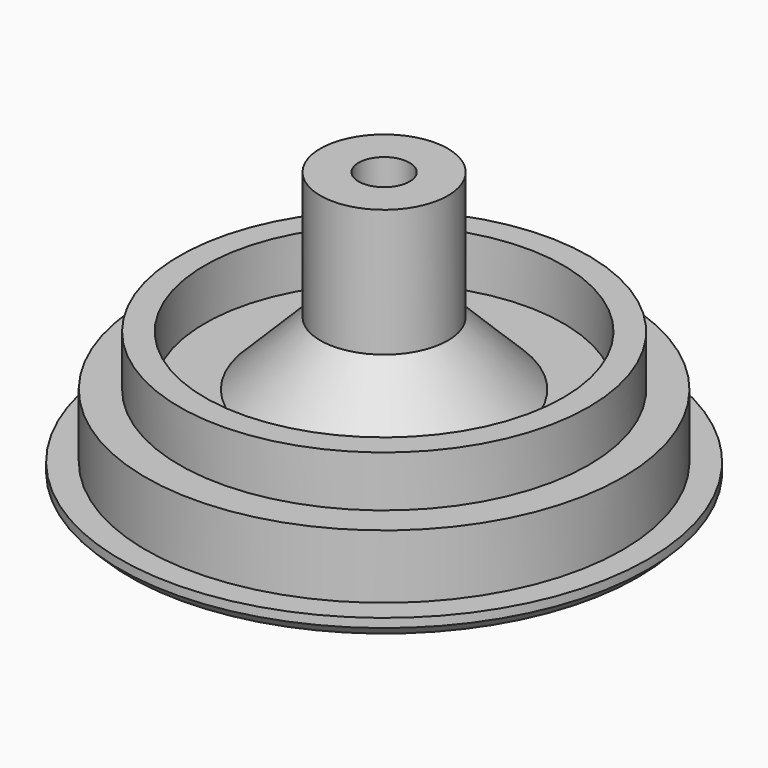
from build123d import *

# Parameters (mm, degrees)
F0_R     = 20.7
F0_R_2   = 18.7
F0_R_3   = 16.05
F0_R_4   = 14.05
F0_R_5   = 5
F0_R_6   = 2
F1_DEPTH = 1.5
F2_DEPTH = 9
F3_DEPTH = 5
F4_SIZE  = 0.8
F5_DEPTH = 20
F6_DEPTH = 5
F7_SIZE  = 1
F8_SIZE  = 5


with BuildPart() as f1:
    # F0 (on Top) → F1 (new body)
    with BuildSketch(Plane.XY):
        Circle(F0_R)
        Circle(F0_R_2, mode=Mode.SUBTRACT)
        Circle(F0_R_2)
        Circle(F0_R_3, mode=Mode.SUBTRACT)
        Circle(F0_R_3)
        Circle(F0_R_4, mode=Mode.SUBTRACT)
        Circle(F0_R_4)
        Circle(F0_R_5, mode=Mode.SUBTRACT)
        Circle(F0_R_5)
        Circle(F0_R_6, mode=Mode.SUBTRACT)
        Circle(F0_R_6)
    extrude(amount=-F1_DEPTH)

    # F0 (on Top) → F2 (join)
    with BuildSketch(Plane.XY):
        Circle(F0_R_3)
        Circle(F0_R_4, mode=Mode.SUBTRACT)
    extrude(amount=F2_DEPTH)

    # F0 (on Top) → F3 (join)
    with BuildSketch(Plane.XY):
        Circle(F0_R_2)
        Circle(F0_R_3, mode=Mode.SUBTRACT)
    extrude(amount=F3_DEPTH)

    # F4
    f4_edges = [f1.edges().sort_by_distance(p)[0] for p in [
        (-20.7, 0, -1.5),
    ]]
    chamfer(f4_edges, length=F4_SIZE)


with BuildPart() as f5:
    # F0 (on Top) → F5 (new body)
    with BuildSketch(Plane.XY):
        Circle(F0_R_5)
        Circle(F0_R_6, mode=Mode.SUBTRACT)
    extrude(amount=F5_DEPTH)

    # F0 (on Top) → F6 (join)
    with BuildSketch(Plane.XY):
        Circle(F0_R_4)
        Circle(F0_R_5, mode=Mode.SUBTRACT)
    extrude(amount=F6_DEPTH)

    # F7
    f7_edges = [f5.edges().sort_by_distance(p)[0] for p in [
        (-14.05, 0, 0),
    ]]
    chamfer(f7_edges, length=F7_SIZE)

    # F8
    f8_edges = [f5.edges().sort_by_distance(p)[0] for p in [
        (-5, 0, 5),
    ]]
    chamfer(f8_edges, length=F8_SIZE)


solid = Compound([f1.part, f5.part])
